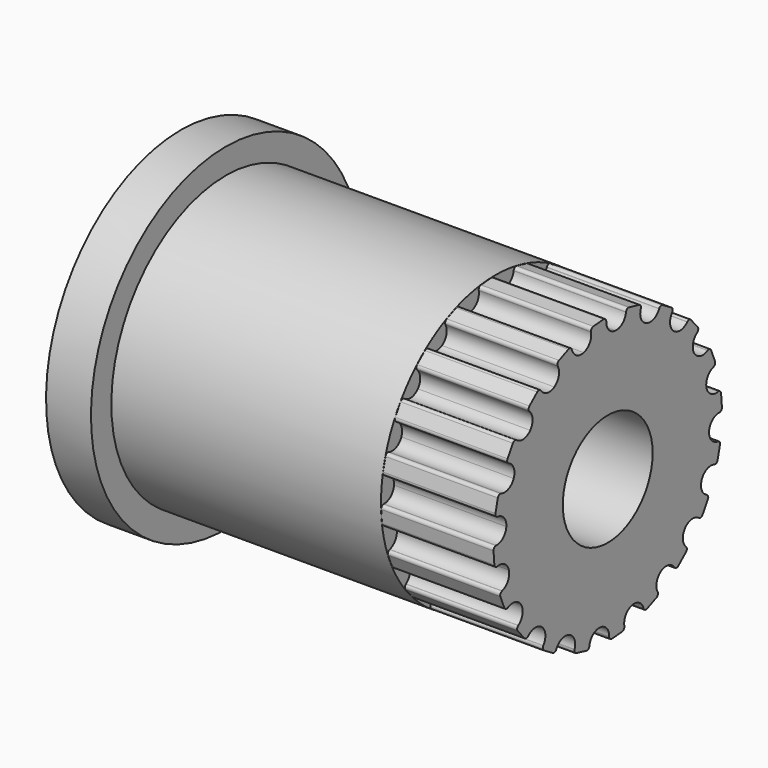
from build123d import *
from build123d import SkipClean  # not in build123d's __all__

# Parameters (mm, degrees)
F0_W     = 12
F0_H     = 3.8661977237
F0_W_2   = 2
F0_H_2   = 1.1338022763
F2_R     = 2.5
F3_DEPTH = 5


with BuildPart() as f1:
    # F0 (on Front) → F1 (revolve)
    with BuildSketch(Plane.XZ):
        with Locations((8, 4.4330988618)):
            Rectangle(F0_W, F0_H)
        with Locations((1, 4.4330988618)):
            Rectangle(F0_W_2, F0_H)
        with Locations((1, 6.9330988618)):
            Rectangle(F0_W_2, F0_H_2)
    revolve(axis=Axis((31.1346538365, 0, 0), (1, 0, 0)))

    # F2 (on face) → F3 (join)
    with BuildSketch(Plane.YZ.offset(14)):
        with BuildLine():
            ThreePointArc((1.0155111033, 6.1225507253), (0.8185107426, 5.7633627955), (0.427864291, 5.6399915636))
            ThreePointArc((0.427864291, 5.6399915636), (0.0602999603, 5.8208826189), (-0.080259854, 6.2056787333))
            Line((-0.080259854, 6.2056787333), (-0.0803901649, 6.2157543541))
            ThreePointArc((-0.0803901649, 6.2157543541), (-0.1261591328, 6.3174944065), (-0.2317565868, 6.353480715))
            Line((-0.2317565868, 6.353480715), (-0.8006133239, 6.3070949427))
            ThreePointArc((-0.8006133239, 6.3070949427), (-0.8989857606, 6.2544765013), (-0.9276675024, 6.1466655818))
            Line((-0.9276675024, 6.1466655818), (-0.9261637709, 6.1367019526))
            ThreePointArc((-0.9261637709, 6.1367019526), (-1.0025270731, 5.734217472), (-1.3359301193, 5.4961680656))
            ThreePointArc((-1.3359301193, 5.4961680656), (-1.7414029814, 5.5546220578), (-1.9939918474, 5.8771495385))
            Line((-1.9939918474, 5.8771495385), (-1.9972293185, 5.886691755))
            ThreePointArc((-1.9972293185, 5.886691755), (-2.0721975988, 5.9693089059), (-2.1837471264, 5.9709025113))
            Line((-2.1837471264, 5.9709025113), (-2.7104280412, 5.7510006212))
            ThreePointArc((-2.7104280412, 5.7510006212), (-2.7877257955, 5.6705587548), (-2.7816883467, 5.5591613317))
            Line((-2.7816883467, 5.5591613317), (-2.7771792822, 5.5501500358))
            ThreePointArc((-2.7771792822, 5.5501500358), (-2.7254305539, 5.1437669897), (-2.9689543815, 4.8143413433))
            ThreePointArc((-2.9689543815, 4.8143413433), (-3.3726452661, 4.7446363883), (-3.7125380257, 4.9733239984))
            Line((-3.7125380257, 4.9733239984), (-3.7185657508, 4.981398752))
            ThreePointArc((-3.7185657508, 4.981398752), (-3.815394926, 5.036805859), (-3.9219772822, 5.003850768))
            Line((-3.9219772822, 5.003850768), (-4.3549271771, 4.6319582892))
            ThreePointArc((-4.3549271771, 4.6319582892), (-4.4035838063, 4.5315672083), (-4.3634181544, 4.4274876374))
            Line((-4.3634181544, 4.4274876374), (-4.3563451357, 4.4203107633))
            ThreePointArc((-4.3563451357, 4.4203107633), (-4.1815499029, 4.0498087557), (-4.3113567029, 3.6612533468))
            ThreePointArc((-4.3113567029, 3.6612533468), (-4.6737495336, 3.4702126513), (-5.0676751154, 3.5826748541))
            Line((-5.0676751154, 3.5826748541), (-5.0759030587, 3.5884917316))
            ThreePointArc((-5.0759030587, 3.5884917316), (-5.1851148144, 3.6112651612), (-5.2762969757, 3.5469872478))
            Line((-5.2762969757, 3.5469872478), (-5.5731356984, 3.0595076072))
            ThreePointArc((-5.5731356984, 3.0595076072), (-5.5883883526, 2.9489942902), (-5.5180261914, 2.8624206051))
            Line((-5.5180261914, 2.8624206051), (-5.5090815748, 2.8577806752))
            ThreePointArc((-5.5090815748, 2.8577806752), (-5.2283500128, 2.559427024), (-5.2317333913, 2.1497763633))
            ThreePointArc((-5.2317333913, 2.1497763633), (-5.5173546328, 1.8561003216), (-5.9267528562, 1.8413285331))
            Line((-5.9267528562, 1.8413285331), (-5.9363756093, 1.8443181381))
            ThreePointArc((-5.9363756093, 1.8443181381), (-6.047279538, 1.8322286681), (-6.114135959, 1.7429199023))
            Line((-6.114135959, 1.7429199023), (-6.2458068672, 1.1875710037))
            ThreePointArc((-6.2458068672, 1.1875710037), (-6.2261625103, 1.0777532641), (-6.1324913784, 1.0171599004))
            Line((-6.1324913784, 1.0171599004), (-6.1225507253, 1.0155111033))
            ThreePointArc((-6.1225507253, 1.0155111033), (-5.7633627955, 0.8185107426), (-5.6399915636, 0.427864291))
            ThreePointArc((-5.6399915636, 0.427864291), (-5.8208826189, 0.0602999603), (-6.2056787333, -0.080259854))
            Line((-6.2056787333, -0.080259854), (-6.2157543541, -0.0803901649))
            ThreePointArc((-6.2157543541, -0.0803901649), (-6.3174944065, -0.1261591328), (-6.353480715, -0.2317565868))
            Line((-6.353480715, -0.2317565868), (-6.3070949427, -0.8006133239))
            ThreePointArc((-6.3070949427, -0.8006133239), (-6.2544765013, -0.8989857606), (-6.1466655818, -0.9276675024))
            Line((-6.1466655818, -0.9276675024), (-6.1367019526, -0.9261637709))
            ThreePointArc((-6.1367019526, -0.9261637709), (-5.734217472, -1.0025270731), (-5.4961680656, -1.3359301193))
            ThreePointArc((-5.4961680656, -1.3359301193), (-5.5546220578, -1.7414029814), (-5.8771495385, -1.9939918474))
            Line((-5.8771495385, -1.9939918474), (-5.886691755, -1.9972293185))
            ThreePointArc((-5.886691755, -1.9972293185), (-5.9693089059, -2.0721975988), (-5.9709025113, -2.1837471264))
            Line((-5.9709025113, -2.1837471264), (-5.7510006212, -2.7104280412))
            ThreePointArc((-5.7510006212, -2.7104280412), (-5.6705587548, -2.7877257955), (-5.5591613317, -2.7816883467))
            Line((-5.5591613317, -2.7816883467), (-5.5501500358, -2.7771792822))
            ThreePointArc((-5.5501500358, -2.7771792822), (-5.1437669897, -2.7254305539), (-4.8143413433, -2.9689543815))
            ThreePointArc((-4.8143413433, -2.9689543815), (-4.7446363883, -3.3726452661), (-4.9733239984, -3.7125380257))
            Line((-4.9733239984, -3.7125380257), (-4.981398752, -3.7185657508))
            ThreePointArc((-4.981398752, -3.7185657508), (-5.036805859, -3.815394926), (-5.003850768, -3.9219772822))
            Line((-5.003850768, -3.9219772822), (-4.6319582892, -4.3549271771))
            ThreePointArc((-4.6319582892, -4.3549271771), (-4.5315672083, -4.4035838063), (-4.4274876374, -4.3634181544))
            Line((-4.4274876374, -4.3634181544), (-4.4203107633, -4.3563451357))
            ThreePointArc((-4.4203107633, -4.3563451357), (-4.0498087557, -4.1815499029), (-3.6612533468, -4.3113567029))
            ThreePointArc((-3.6612533468, -4.3113567029), (-3.4702126513, -4.6737495336), (-3.5826748541, -5.0676751154))
            Line((-3.5826748541, -5.0676751154), (-3.5884917316, -5.0759030587))
            ThreePointArc((-3.5884917316, -5.0759030587), (-3.6112651612, -5.1851148144), (-3.5469872478, -5.2762969757))
            Line((-3.5469872478, -5.2762969757), (-3.0595076072, -5.5731356984))
            ThreePointArc((-3.0595076072, -5.5731356984), (-2.9489942902, -5.5883883526), (-2.8624206051, -5.5180261914))
            Line((-2.8624206051, -5.5180261914), (-2.8577806752, -5.5090815748))
            ThreePointArc((-2.8577806752, -5.5090815748), (-2.559427024, -5.2283500128), (-2.1497763633, -5.2317333913))
            ThreePointArc((-2.1497763633, -5.2317333913), (-1.8561003216, -5.5173546328), (-1.8413285331, -5.9267528562))
            Line((-1.8413285331, -5.9267528562), (-1.8443181381, -5.9363756093))
            ThreePointArc((-1.8443181381, -5.9363756093), (-1.8322286681, -6.047279538), (-1.7429199023, -6.114135959))
            Line((-1.7429199023, -6.114135959), (-1.1875710037, -6.2458068672))
            ThreePointArc((-1.1875710037, -6.2458068672), (-1.0777532641, -6.2261625103), (-1.0171599004, -6.1324913784))
            Line((-1.0171599004, -6.1324913784), (-1.0155111033, -6.1225507253))
            ThreePointArc((-1.0155111033, -6.1225507253), (-0.8185107426, -5.7633627955), (-0.427864291, -5.6399915636))
            ThreePointArc((-0.427864291, -5.6399915636), (-0.0602999603, -5.8208826189), (0.080259854, -6.2056787333))
            Line((0.080259854, -6.2056787333), (0.0803901649, -6.2157543541))
            ThreePointArc((0.0803901649, -6.2157543541), (0.1261591328, -6.3174944065), (0.2317565868, -6.353480715))
            Line((0.2317565868, -6.353480715), (0.8006133239, -6.3070949427))
            ThreePointArc((0.8006133239, -6.3070949427), (0.8989857606, -6.2544765013), (0.9276675024, -6.1466655818))
            Line((0.9276675024, -6.1466655818), (0.9261637709, -6.1367019526))
            ThreePointArc((0.9261637709, -6.1367019526), (1.0025270731, -5.734217472), (1.3359301193, -5.4961680656))
            ThreePointArc((1.3359301193, -5.4961680656), (1.7414029814, -5.5546220578), (1.9939918474, -5.8771495385))
            Line((1.9939918474, -5.8771495385), (1.9972293185, -5.886691755))
            ThreePointArc((1.9972293185, -5.886691755), (2.0721975988, -5.9693089059), (2.1837471264, -5.9709025113))
            Line((2.1837471264, -5.9709025113), (2.7104280412, -5.7510006212))
            ThreePointArc((2.7104280412, -5.7510006212), (2.7877257955, -5.6705587548), (2.7816883467, -5.5591613317))
            Line((2.7816883467, -5.5591613317), (2.7771792822, -5.5501500358))
            ThreePointArc((2.7771792822, -5.5501500358), (2.7254305539, -5.1437669897), (2.9689543815, -4.8143413433))
            ThreePointArc((2.9689543815, -4.8143413433), (3.3726452661, -4.7446363883), (3.7125380257, -4.9733239984))
            Line((3.7125380257, -4.9733239984), (3.7185657508, -4.981398752))
            ThreePointArc((3.7185657508, -4.981398752), (3.815394926, -5.036805859), (3.9219772822, -5.003850768))
            Line((3.9219772822, -5.003850768), (4.3549271771, -4.6319582892))
            ThreePointArc((4.3549271771, -4.6319582892), (4.4035838063, -4.5315672083), (4.3634181544, -4.4274876374))
            Line((4.3634181544, -4.4274876374), (4.3563451357, -4.4203107633))
            ThreePointArc((4.3563451357, -4.4203107633), (4.1815499029, -4.0498087557), (4.3113567029, -3.6612533468))
            ThreePointArc((4.3113567029, -3.6612533468), (4.6737495336, -3.4702126513), (5.0676751154, -3.5826748541))
            Line((5.0676751154, -3.5826748541), (5.0759030587, -3.5884917316))
            ThreePointArc((5.0759030587, -3.5884917316), (5.1851148144, -3.6112651612), (5.2762969757, -3.5469872478))
            Line((5.2762969757, -3.5469872478), (5.5731356984, -3.0595076072))
            ThreePointArc((5.5731356984, -3.0595076072), (5.5883883526, -2.9489942902), (5.5180261914, -2.8624206051))
            Line((5.5180261914, -2.8624206051), (5.5090815748, -2.8577806752))
            ThreePointArc((5.5090815748, -2.8577806752), (5.2283500128, -2.559427024), (5.2317333913, -2.1497763633))
            ThreePointArc((5.2317333913, -2.1497763633), (5.5173546328, -1.8561003216), (5.9267528562, -1.8413285331))
            Line((5.9267528562, -1.8413285331), (5.9363756093, -1.8443181381))
            ThreePointArc((5.9363756093, -1.8443181381), (6.047279538, -1.8322286681), (6.114135959, -1.7429199023))
            Line((6.114135959, -1.7429199023), (6.2458068672, -1.1875710037))
            ThreePointArc((6.2458068672, -1.1875710037), (6.2261625103, -1.0777532641), (6.1324913784, -1.0171599004))
            Line((6.1324913784, -1.0171599004), (6.1225507253, -1.0155111033))
            ThreePointArc((6.1225507253, -1.0155111033), (5.7633627955, -0.8185107426), (5.6399915636, -0.427864291))
            ThreePointArc((5.6399915636, -0.427864291), (5.8208826189, -0.0602999603), (6.2056787333, 0.080259854))
            Line((6.2056787333, 0.080259854), (6.2157543541, 0.0803901649))
            ThreePointArc((6.2157543541, 0.0803901649), (6.3174944065, 0.1261591328), (6.353480715, 0.2317565868))
            Line((6.353480715, 0.2317565868), (6.3070949427, 0.8006133239))
            ThreePointArc((6.3070949427, 0.8006133239), (6.2544765013, 0.8989857606), (6.1466655818, 0.9276675024))
            Line((6.1466655818, 0.9276675024), (6.1367019526, 0.9261637709))
            ThreePointArc((6.1367019526, 0.9261637709), (5.734217472, 1.0025270731), (5.4961680656, 1.3359301193))
            ThreePointArc((5.4961680656, 1.3359301193), (5.5546220578, 1.7414029814), (5.8771495385, 1.9939918474))
            Line((5.8771495385, 1.9939918474), (5.886691755, 1.9972293185))
            ThreePointArc((5.886691755, 1.9972293185), (5.9693089059, 2.0721975988), (5.9709025113, 2.1837471264))
            Line((5.9709025113, 2.1837471264), (5.7510006212, 2.7104280412))
            ThreePointArc((5.7510006212, 2.7104280412), (5.6705587548, 2.7877257955), (5.5591613317, 2.7816883467))
            Line((5.5591613317, 2.7816883467), (5.5501500358, 2.7771792822))
            ThreePointArc((5.5501500358, 2.7771792822), (5.1437669897, 2.7254305539), (4.8143413433, 2.9689543815))
            ThreePointArc((4.8143413433, 2.9689543815), (4.7446363883, 3.3726452661), (4.9733239984, 3.7125380257))
            Line((4.9733239984, 3.7125380257), (4.981398752, 3.7185657508))
            ThreePointArc((4.981398752, 3.7185657508), (5.036805859, 3.815394926), (5.003850768, 3.9219772822))
            Line((5.003850768, 3.9219772822), (4.6319582892, 4.3549271771))
            ThreePointArc((4.6319582892, 4.3549271771), (4.5315672083, 4.4035838063), (4.4274876374, 4.3634181544))
            Line((4.4274876374, 4.3634181544), (4.4203107633, 4.3563451357))
            ThreePointArc((4.4203107633, 4.3563451357), (4.0498087557, 4.1815499029), (3.6612533468, 4.3113567029))
            ThreePointArc((3.6612533468, 4.3113567029), (3.4702126513, 4.6737495336), (3.5826748541, 5.0676751154))
            Line((3.5826748541, 5.0676751154), (3.5884917316, 5.0759030587))
            ThreePointArc((3.5884917316, 5.0759030587), (3.6112651612, 5.1851148144), (3.5469872478, 5.2762969757))
            Line((3.5469872478, 5.2762969757), (3.0595076072, 5.5731356984))
            ThreePointArc((3.0595076072, 5.5731356984), (2.9489942902, 5.5883883526), (2.8624206051, 5.5180261914))
            Line((2.8624206051, 5.5180261914), (2.8577806752, 5.5090815748))
            ThreePointArc((2.8577806752, 5.5090815748), (2.559427024, 5.2283500128), (2.1497763633, 5.2317333913))
            ThreePointArc((2.1497763633, 5.2317333913), (1.8561003216, 5.5173546328), (1.8413285331, 5.9267528562))
            Line((1.8413285331, 5.9267528562), (1.8443181381, 5.9363756093))
            ThreePointArc((1.8443181381, 5.9363756093), (1.8322286681, 6.047279538), (1.7429199023, 6.114135959))
            Line((1.7429199023, 6.114135959), (1.1875710037, 6.2458068672))
            ThreePointArc((1.1875710037, 6.2458068672), (1.0777532641, 6.2261625103), (1.0171599004, 6.1324913784))
            Line((1.0171599004, 6.1324913784), (1.0155111033, 6.1225507253))
        make_face()
        Circle(F2_R, mode=Mode.SUBTRACT)
    with SkipClean():  # cleaning this boolean's faces spoils the solid; the shape is the same uncleaned
        extrude(amount=F3_DEPTH)


solid = f1.part
